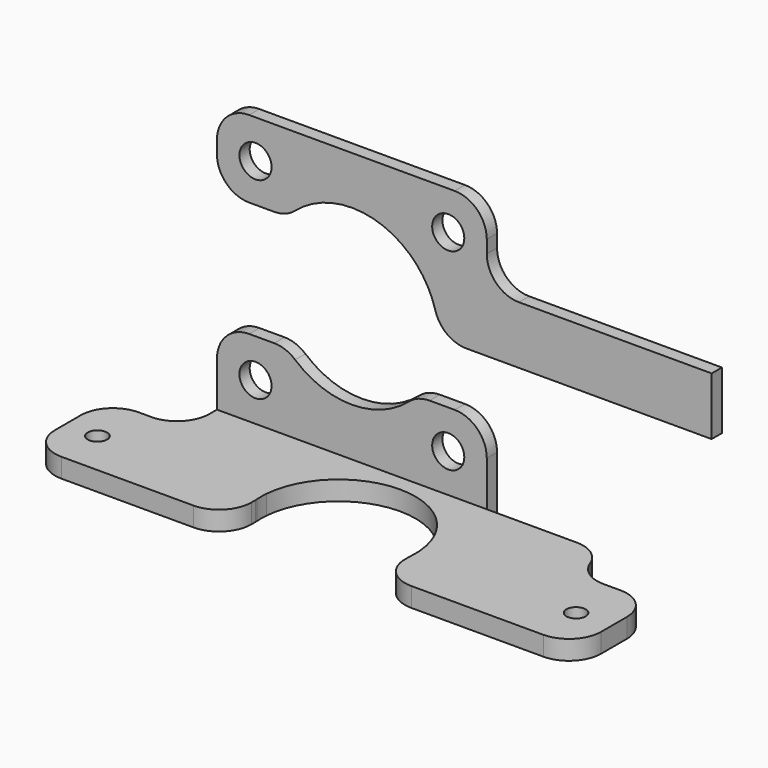
from build123d import *

# Parameters (mm, degrees)
F0_W        = 12
F0_H        = 15
F0_W_2      = 42
F0_H_2      = 2
F0_W_3      = 17
F0_H_3      = 6.5
F1_DEPTH    = 3
F2_D        = 3
F2_DEPTH    = 10
F2_TIP      = 0.9012909285
F3_DEPTH    = 45
F4_R        = 2.5
F5_DEPTH    = 25
F6_T1_DEPTH = 3
F6_T3_DEPTH = 28
F6_T5_DEPTH = 27
F6_T7_DEPTH = 12.1554036185
F6_T9_DEPTH = 3.9527148617
F6_S1_F1_R  = 5
F6_S1_F2_R  = 5
F6_S1_F3_R  = 5
F6_S1_F4_R  = 5
F6_S1_F5_R  = 5
F7_R        = 5
F4_W        = 35
F4_H        = 9
F8_DEPTH    = 2
F9_R        = 5


# Not quite as in the source:
# - a fillet or chamfer that OpenCascade refuses, or shapes differently, is made with other operations: its cross-section is extruded or revolved along the edge and cut away or added


with BuildPart() as f1:
    # F0 (on Top) → F1 (new body)
    with BuildSketch(Plane.XY):
        with Locations((-36.5, -0.5)):
            Rectangle(F0_W, F0_H)
        with Locations((36.5, -0.5)):
            Rectangle(F0_W, F0_H)
        with Locations((-9.5, 14.5)):
            Rectangle(F0_W_2, F0_H_2)
        with BuildLine():
            Line((-30.5, 13.5), (-30.5, 7))
            Line((-30.5, 7), (-30.5, -8))
            Line((-30.5, -8), (-11.9582607431, -8))
            Line((-11.9582607431, -8), (-11.9582607431, -2))
            ThreePointArc((-11.9582607431, -2), (-12, -1), (-11.9582607431, 0))
            ThreePointArc((-11.9582607431, 0), (0, 11), (11.9582607431, 0))
            ThreePointArc((11.9582607431, 0), (11.9895606449, -0.4995646481), (12, -1))
            ThreePointArc((12, -1), (11.9895606449, -1.5004353519), (11.9582607431, -2))
            Line((11.9582607431, -2), (11.9582607431, -8))
            Line((11.9582607431, -8), (30.5, -8))
            Line((30.5, -8), (30.5, 7))
            Line((30.5, 7), (13.5, 7))
            Line((13.5, 7), (13.5, 13.5))
            Line((13.5, 13.5), (11.5, 13.5))
            Line((11.5, 13.5), (-30.5, 13.5))
        make_face()
        with Locations((22, 10.25)):
            Rectangle(F0_W_3, F0_H_3)
    extrude(amount=F1_DEPTH)

    # F2
    with Locations(Plane(origin=(0, 0, 0), x_dir=(1, 0, 0), z_dir=(0, 0, -1))):
        with Locations((-37.5, 1), (37, 1)):
            Hole(F2_D / 2, depth=F2_DEPTH)
            with Locations((0, 0, -(F2_DEPTH + F2_TIP / 2))):  # 118° drill point
                Cone(0, F2_D / 2, F2_TIP, mode=Mode.SUBTRACT)

    # F0 (on Top) → F3 (join)
    with BuildSketch(Plane.XY):
        with Locations((-9.5, 14.5)):
            Rectangle(F0_W_2, F0_H_2)
    extrude(amount=F3_DEPTH)

    # F4 (on face) → F5 (cut)
    with BuildSketch(Plane.XZ.offset(-13.5)):
        with Locations((-24.5, 39)):
            Circle(F4_R)
        with Locations((5.5, 39)):
            Circle(F4_R)
        with Locations((-24.5, 9)):
            Circle(F4_R)
        with Locations((5.5, 9)):
            Circle(F4_R)
        with BuildLine():
            ThreePointArc((0.5623058987, 15), (3.111326846, 19.1829017881), (4, 24))
            ThreePointArc((4, 24), (3.111326846, 28.8170982119), (0.5623058987, 33))
            ThreePointArc((0.5623058987, 33), (0.045941546, 33.545941546), (-0.5, 34.0623058987))
            ThreePointArc((-0.5, 34.0623058987), (-9.5, 37.5), (-18.5, 34.0623058987))
            ThreePointArc((-18.5, 34.0623058987), (-19.045941546, 33.545941546), (-19.5623058987, 33))
            ThreePointArc((-19.5623058987, 33), (-22.111326846, 28.8170982119), (-23, 24))
            ThreePointArc((-23, 24), (-22.111326846, 19.1829017881), (-19.5623058987, 15))
            ThreePointArc((-19.5623058987, 15), (-9.5, 10.5), (0.5623058987, 15))
        make_face()
        with BuildLine():
            Line((-30.5, 15), (-19.5623058987, 15))
            ThreePointArc((-19.5623058987, 15), (-22.111326846, 19.1829017881), (-23, 24))
            Line((-23, 24), (-30.5, 24))
            Line((-30.5, 24), (-30.5, 15))
        make_face()
        with BuildLine():
            Line((11.5, 24), (4, 24))
            ThreePointArc((4, 24), (3.111326846, 19.1829017881), (0.5623058987, 15))
            Line((0.5623058987, 15), (11.5, 15))
            Line((11.5, 15), (11.5, 24))
        make_face()
        with BuildLine():
            Line((-30.5, 24), (-23, 24))
            ThreePointArc((-23, 24), (-22.111326846, 28.8170982119), (-19.5623058987, 33))
            Line((-19.5623058987, 33), (-30.5, 33))
            Line((-30.5, 33), (-30.5, 24))
        make_face()
    extrude(amount=-F5_DEPTH, mode=Mode.SUBTRACT)

    # F6: fillet of radius 5 on 14 edges, made by hand

    # F6_s2 → F6_t1 (join)
    with BuildSketch(Plane.XY):
        with BuildLine():
            ThreePointArc((-35.5, 7), (-31.9644660941, 8.4644660941), (-30.5, 12))
            Line((-30.5, 12), (-30.5, 7))
            Line((-30.5, 7), (-35.5, 7))
        make_face()
    extrude(amount=F6_T1_DEPTH)

    # F6_s4 → F6_t3 (cut)
    with BuildSketch(Plane.XY.offset(-12.5)):
        with BuildLine():
            ThreePointArc((-42.5, -3), (-41.0355339059, -6.5355339059), (-37.5, -8))
            Line((-37.5, -8), (-42.5, -8))
            Line((-42.5, -8), (-42.5, -3))
        make_face()
        with BuildLine():
            ThreePointArc((-37.5, 7), (-41.0355339059, 5.5355339059), (-42.5, 2))
            Line((-42.5, 2), (-42.5, 7))
            Line((-42.5, 7), (-37.5, 7))
        make_face()
        with BuildLine():
            ThreePointArc((42.5, 2), (41.0355339059, 5.5355339059), (37.5, 7))
            Line((37.5, 7), (42.5, 7))
            Line((42.5, 7), (42.5, 2))
        make_face()
        with BuildLine():
            ThreePointArc((37.5, -8), (41.0355339059, -6.5355339059), (42.5, -3))
            Line((42.5, -3), (42.5, -8))
            Line((42.5, -8), (37.5, -8))
        make_face()
        with BuildLine():
            ThreePointArc((30.5, 8.5), (29.0355339059, 12.0355339059), (25.5, 13.5))
            Line((25.5, 13.5), (30.5, 13.5))
            Line((30.5, 13.5), (30.5, 8.5))
        make_face()
        with BuildLine():
            ThreePointArc((-16.9582607431, -8), (-13.4227268372, -6.5355339059), (-11.9582607431, -3))
            Line((-11.9582607431, -3), (-11.9582607431, -8))
            Line((-11.9582607431, -8), (-16.9582607431, -8))
        make_face()
        with BuildLine():
            ThreePointArc((11.9582607431, -3), (13.4227268372, -6.5355339059), (16.9582607431, -8))
            Line((16.9582607431, -8), (11.9582607431, -8))
            Line((11.9582607431, -8), (11.9582607431, -3))
        make_face()
    extrude(amount=F6_T3_DEPTH, mode=Mode.SUBTRACT)

    # F6_s6 → F6_t5 (cut)
    with BuildSketch(Plane.XZ.offset(-28)):
        with BuildLine():
            ThreePointArc((-30.5, 10), (-29.0355339059, 13.5355339059), (-25.5, 15))
            Line((-25.5, 15), (-30.5, 15))
            Line((-30.5, 15), (-30.5, 10))
        make_face()
        with BuildLine():
            ThreePointArc((11.5, 10), (10.0355339059, 13.5355339059), (6.5, 15))
            Line((6.5, 15), (11.5, 15))
            Line((11.5, 15), (11.5, 10))
        make_face()
    extrude(amount=F6_T5_DEPTH, mode=Mode.SUBTRACT)

    # F6_s8 → F6_t7 (cut)
    with BuildSketch(Plane.XZ.offset(-20.5777018093)):
        with BuildLine():
            ThreePointArc((-21.5933866224, 15), (-19.8496720413, 14.6860921309), (-18.3249037515, 13.7837837838))
            ThreePointArc((-18.3249037515, 13.7837837838), (-18.9631637186, 14.3719922915), (-19.5623058987, 15))
            Line((-19.5623058987, 15), (-21.5933866224, 15))
        make_face()
        with BuildLine():
            ThreePointArc((2.5933866224, 15), (0.8496720413, 14.6860921309), (-0.6750962485, 13.7837837838))
            ThreePointArc((-0.6750962485, 13.7837837838), (-0.0368362814, 14.3719922915), (0.5623058987, 15))
            Line((0.5623058987, 15), (2.5933866224, 15))
        make_face()
    extrude(amount=F6_T7_DEPTH, mode=Mode.SUBTRACT)

    # F6_s10 → F6_t9 (cut)
    with BuildSketch(Plane.XY.offset(-0.4763574308)):
        with BuildLine():
            ThreePointArc((-11.9582607431, -2.1905429723), (-11.9613307486, -2.0153555582), (-11.9705369951, -1.8403832746))
            ThreePointArc((-11.9705369951, -1.8403832746), (-11.9646650465, -1.9202121092), (-11.9582607431, -2))
            Line((-11.9582607431, -2), (-11.9582607431, -2.1905429723))
        make_face()
        with BuildLine():
            ThreePointArc((11.9705369951, -1.8403832746), (11.9613307486, -2.0153555582), (11.9582607431, -2.1905429723))
            Line((11.9582607431, -2.1905429723), (11.9582607431, -2))
            ThreePointArc((11.9582607431, -2), (11.9646650465, -1.9202121092), (11.9705369951, -1.8403832746))
        make_face()
    extrude(amount=F6_T9_DEPTH, mode=Mode.SUBTRACT)

    # F6#s1: fillet of radius 5 on 5 edges, made by hand

    # F6_s1_f1
    f6_s1_f1_edges = [f1.edges().sort_by_distance(p)[0] for p in [
        (-30.5, 14.5, 33),
    ]]
    fillet(f6_s1_f1_edges, radius=F6_S1_F1_R)

    # F6_s1_f2
    f6_s1_f2_edges = [f1.edges().sort_by_distance(p)[0] for p in [
        (-30.5, 14.5, 45),
    ]]
    fillet(f6_s1_f2_edges, radius=F6_S1_F2_R)

    # F6_s1_f3
    f6_s1_f3_edges = [f1.edges().sort_by_distance(p)[0] for p in [
        (-19.5623058987, 14.5, 33),
    ]]
    fillet(f6_s1_f3_edges, radius=F6_S1_F3_R)

    # F6_s1_f4
    f6_s1_f4_edges = [f1.edges().sort_by_distance(p)[0] for p in [
        (11.5, 14.5, 45),
    ]]
    fillet(f6_s1_f4_edges, radius=F6_S1_F4_R)

    # F6_s1_f5
    f6_s1_f5_edges = [f1.edges().sort_by_distance(p)[0] for p in [
        (4, 14.5, 24),
    ]]
    fillet(f6_s1_f5_edges, radius=F6_S1_F5_R)

    # F7
    f7_edges = [f1.edges().sort_by_distance(p)[0] for p in [
        (30.5, 7, 1.5),
    ]]
    fillet(f7_edges, radius=F7_R)

    # F4 (on face) → F8 (join)
    with BuildSketch(Plane.XZ.offset(-13.5)):
        with Locations((29, 28.5)):
            Rectangle(F4_W, F4_H)
    extrude(amount=-F8_DEPTH)

    # F9
    f9_edges = [f1.edges().sort_by_distance(p)[0] for p in [
        (11.5, 14.5, 33),
    ]]
    fillet(f9_edges, radius=F9_R)


solid = f1.part
